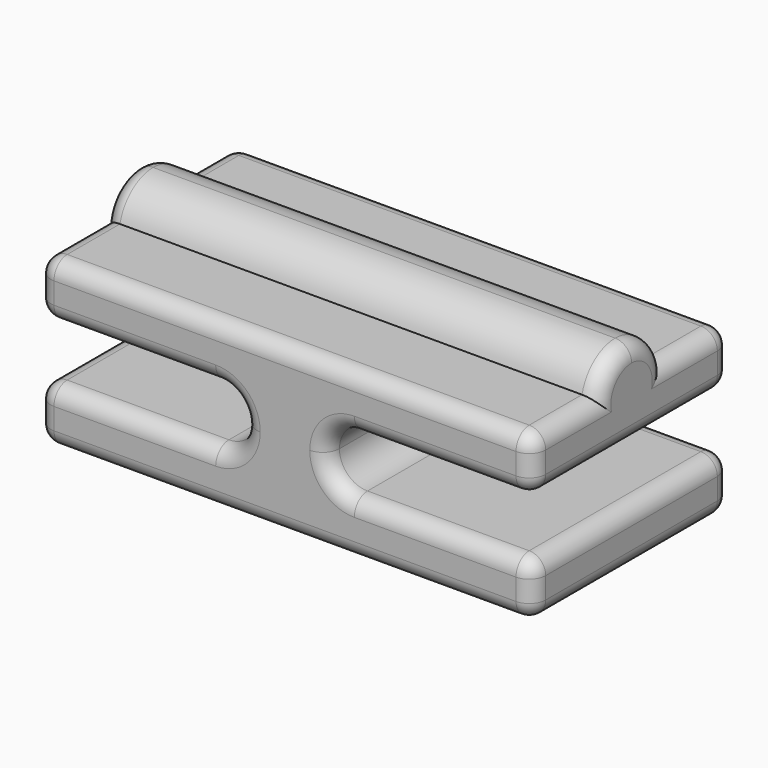
from build123d import *

# Parameters (mm, degrees)
F0_W        = 15
F0_H        = 15
F1_DEPTH    = 10
F2_W        = 15
F2_H        = 3.4
F3_DEPTH    = 12.5
F4_R        = 1.69999
F6_W        = 5
F6_H        = 2
F7_DEPTH    = 30
F8_T1_DEPTH = 42.6491106407
F9_R        = 1


# Not quite as in the source:
# - a fillet or chamfer that OpenCascade refuses, or shapes differently, is made with other operations: its cross-section is extruded or revolved along the edge and cut away or added
# - a fillet or chamfer is up to 0.001 mm smaller than in the source, because OpenCascade refuses the exact size


with BuildPart() as f1:
    # F0 (on Top) → F1 (new body)
    with BuildSketch(Plane.XY):
        with Locations((7.5, 7.5)):
            Rectangle(F0_W, F0_H)
    extrude(amount=F1_DEPTH)

    # F2 (on face) → F3 (cut)
    with BuildSketch(Plane.YZ.offset(15)):
        with Locations((7.5, 5)):
            Rectangle(F2_W, F2_H)
    extrude(amount=-F3_DEPTH, mode=Mode.SUBTRACT)

    # F4 (radius 1.7 in the source; OpenCascade refuses exactly that, so slightly less here)
    f4_edges = [f1.edges().sort_by_distance(p)[0] for p in [
        (2.5, 7.5, 3.3),
        (2.5, 7.5, 6.7),
    ]]
    fillet(f4_edges, radius=F4_R)

    # F5: F1 across face


with BuildPart() as f1_1:
    add(f1.part)
    add(f1.part.mirror(Plane(origin=(0, 7.5, 5), x_dir=(0, -1, 0), z_dir=(-1, 0, 0))))

    # F6 (on face) → F7 (join, through all)
    with BuildSketch(Plane.YZ.offset(15)):
        with Locations((7.5, 11)):
            Rectangle(F6_W, F6_H)
    extrude(amount=-F7_DEPTH)

    # F8: fillet of radius 2.6 on 2 edges, made by hand

    # F8_s2 → F8_t1 (cut)
    with BuildSketch(Plane.YZ.offset(-21.3245553203)):
        with BuildLine():
            ThreePointArc((5, 10), (5.9173705785, 11.4396078054), (7.5298221281, 12))
            Line((7.5298221281, 12), (5, 12))
            Line((5, 12), (5, 10))
        make_face()
        with BuildLine():
            ThreePointArc((10, 10), (9.0826294215, 11.4396078054), (7.4701778719, 12))
            Line((7.4701778719, 12), (10, 12))
            Line((10, 12), (10, 10))
        make_face()
    extrude(amount=F8_T1_DEPTH, mode=Mode.SUBTRACT)

    # F9
    f9_edges = [f1_1.edges().sort_by_distance(p)[0] for p in [
        (-9.599995, 0, 3.3),
        (9.599995, 0, 3.3),
        (-15, 7.5, 3.3),
        (-15, 7.5, 0),
        (-15, 7.5, 6.7),
        (0, 15, 0),
        (-9.599995, 15, 3.3),
        (9.599995, 15, 6.7),
        (15, 7.5, 0),
        (15, 7.5, 6.7),
        (15, 7.5, 3.3),
        (0, 0, 0),
        (-15, 15, 1.65),
        (15, 15, 1.65),
        (15, 0, 1.65),
        (-15, 0, 1.65),
        (15, 5.9057, 11.430327),
        (15, 2.5, 10),
        (15, 12.5, 10),
        (-15, 2.5, 10),
        (-15, 12.5, 10),
        (0, 0, 10),
        (-15, 0, 8.35),
        (15, 0, 8.35),
        (-15, 15, 8.35),
        (15, 15, 8.35),
        (15, 9.0943, 11.430327),
        (-15, 9.0943, 11.430327),
        (-15, 5.9057, 11.430327),
        (0, 15, 10),
        (-9.599995, 15, 6.7),
        (-2.997916, 15, 6.202084),
        (-2.5, 15, 5),
        (-2.997916, 15, 3.797916),
        (9.599995, 15, 3.3),
        (2.997916, 15, 3.797916),
        (2.5, 15, 5),
        (2.997916, 15, 6.202084),
        (9.599995, 0, 6.7),
        (-9.599995, 0, 6.7),
        (-2.997916, 0, 6.202084),
        (-2.5, 0, 5),
        (-2.997916, 0, 3.797916),
        (2.997916, 0, 3.797916),
        (2.5, 0, 5),
        (2.997916, 0, 6.202084),
    ]]
    fillet(f9_edges, radius=F9_R)


solid = f1_1.part
